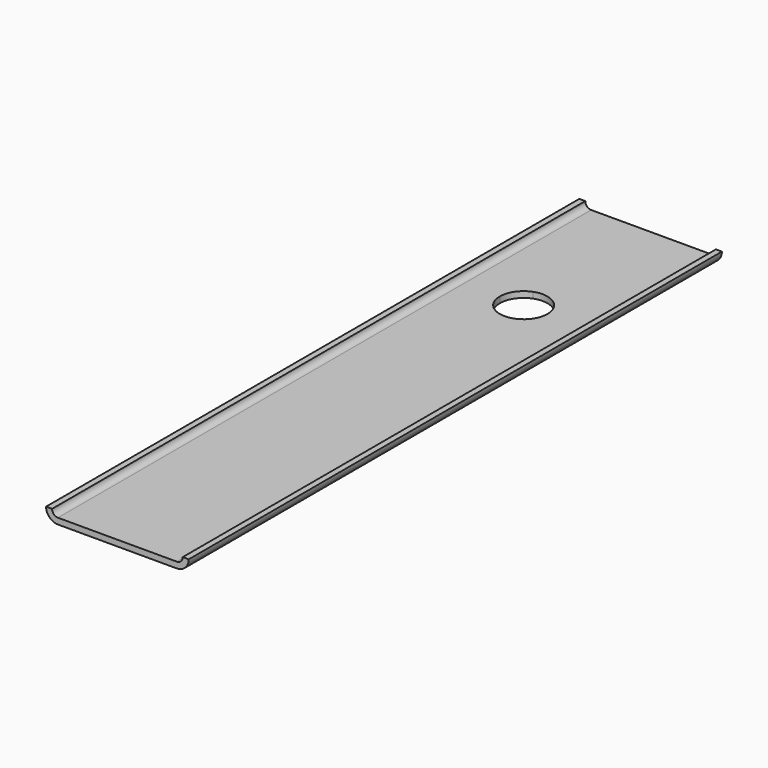
from build123d import *

# Parameters (mm, degrees)
F1_START = 12.7
F1_DEPTH = 88.9
F3_DEPTH = 0.8001


# Not quite as in the source:
# - a feature names something its author has since deleted; it is built from what else it names


with BuildPart() as f1:
    # F0 (on Front) → F1 (new body)
    with BuildSketch(Plane.XZ.offset(F1_START)):
        with BuildLine():
            ThreePointArc((-1.5875, 1.5875), (-1.1225320151, 0.4649679849), (0, 0))
            Line((0, 0), (15.8496, 0))
            ThreePointArc((15.8496, 0), (16.9721320151, 0.4649679849), (17.4371, 1.5875))
            Line((17.4371, 1.5875), (16.637, 1.5875))
            ThreePointArc((16.637, 1.5875), (16.4063758795, 1.0307241205), (15.8496, 0.8001))
            Line((15.8496, 0.8001), (7.9248, 0.8001))
            Line((7.9248, 0.8001), (0, 0.8001))
            ThreePointArc((0, 0.8001), (-0.5567758795, 1.0307241205), (-0.7874, 1.5875))
            Line((-0.7874, 1.5875), (-1.5875, 1.5875))
        make_face()
    extrude(amount=F1_DEPTH)

    # F2 (on face) → F3 (cut, through all)
    with BuildSketch(Plane.XY.offset(0.8001)):
        with BuildLine():
            Line((4.7498, -33.8666666667), (7.9248, -33.8666666667))
            Line((7.9248, -33.8666666667), (6.8115473336, -30.8932353995))
            ThreePointArc((6.8115473336, -30.8932353995), (5.3156619991, -32.0575166198), (4.7498, -33.8666666667))
        make_face()
        with BuildLine():
            Line((7.9248, -33.8666666667), (11.0998, -33.8666666667))
            ThreePointArc((11.0998, -33.8666666667), (9.7339500469, -31.2575286657), (6.8115473336, -30.8932353995))
            Line((6.8115473336, -30.8932353995), (7.9248, -33.8666666667))
        make_face()
        with BuildLine():
            ThreePointArc((4.7498, -33.8666666667), (7.9248, -37.0416666667), (11.0998, -33.8666666667))
            Line((11.0998, -33.8666666667), (7.9248, -33.8666666667))
            Line((7.9248, -33.8666666667), (4.7498, -33.8666666667))
        make_face()
    extrude(amount=-F3_DEPTH, mode=Mode.SUBTRACT)


solid = f1.part
